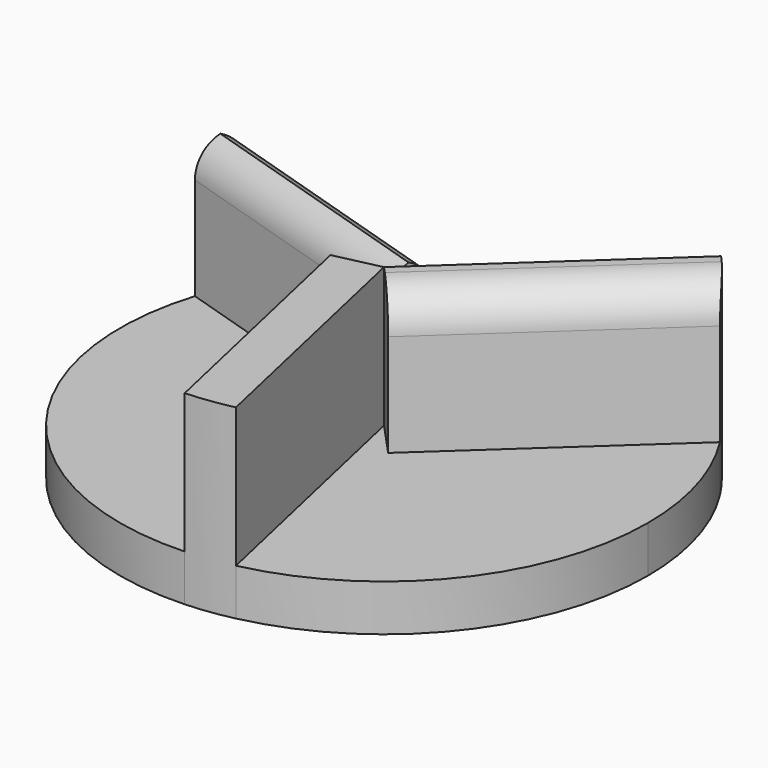
from build123d import *

# Parameters (mm, degrees)
F1_DEPTH      = 25.4
F2_DEPTH      = 6.35
F3_T1_DEPTH   = 61.4532364119
F3_T3_DEPTH   = 60.8896232126
F3_2_T1_DEPTH = 60.8896232126


# Not quite as in the source:
# - a fillet or chamfer that OpenCascade refuses, or shapes differently, is made with other operations: its cross-section is extruded or revolved along the edge and cut away or added


with BuildPart() as f1:
    # F0 (on Top) → F1 (new body)
    with BuildSketch(Plane.XY):
        with BuildLine():
            Line((-34.4173737851, 10.7368634857), (0, 0))
            Line((0, 0), (1.891066931, 6.0618780805))
            Line((1.891066931, 6.0618780805), (-31.9882667756, 16.6308942775))
            ThreePointArc((-31.9882667756, 16.6308942775), (-33.3333492813, 13.737673801), (-34.4173737851, 10.7368634857))
        make_face()
    extrude(amount=F1_DEPTH)

    # F3: fillet of radius 5.08 on 2 edges, made by hand

    # F3_s2 → F3_t1 (cut)
    with BuildSketch(Plane(origin=(-46.541129946, 14.5189973478, 0), x_dir=(0, 0, 1), z_dir=(0.9546264694, -0.2978058159, 0))):
        with BuildLine():
            ThreePointArc((20.32, 0), (23.9121024484, -1.4878975516), (25.4, -5.08))
            Line((25.4, -5.08), (25.4, 0))
            Line((25.4, 0), (20.32, 0))
        make_face()
    extrude(amount=F3_T1_DEPTH, mode=Mode.SUBTRACT)

    # F3_s4 → F3_t3 (cut)
    with BuildSketch(Plane(origin=(12.1237561609, -3.782133862, 0), x_dir=(0, 0, 1), z_dir=(-0.9546264694, 0.2978058159, 0))):
        with BuildLine():
            ThreePointArc((20.32, 6.35), (23.9121024484, 4.8621024484), (25.4, 1.27))
            Line((25.4, 1.27), (25.4, 6.35))
            Line((25.4, 6.35), (20.32, 6.35))
        make_face()
    extrude(amount=F3_T3_DEPTH, mode=Mode.SUBTRACT)


with BuildPart() as f1b:
    # F0 (on Top) → F1, piece 2 (new body)
    with BuildSketch(Plane.XY):
        with BuildLine():
            ThreePointArc((1.5913564558, -36.0180987894), (4.7695001401, -35.7363641714), (7.9102903569, -35.1747517723))
            Line((7.9102903569, -35.1747517723), (0, 0))
            Line((0, 0), (-6.1952738778, -1.3932270377))
            Line((-6.1952738778, -1.3932270377), (1.5913564558, -36.0180987894))
        make_face()
    extrude(amount=F1_DEPTH)


with BuildPart() as f1c:
    # F0 (on Top) → F1, piece 3 (new body)
    with BuildSketch(Plane.XY):
        with BuildLine():
            Line((4.3042069468, -4.6686510427), (30.3969103198, 19.3872045119))
            ThreePointArc((30.3969103198, 19.3872045119), (28.5638491413, 21.9986903703), (26.5070834282, 24.4378882866))
            Line((26.5070834282, 24.4378882866), (0, 0))
            Line((0, 0), (4.3042069468, -4.6686510427))
        make_face()
    extrude(amount=F1_DEPTH)

    # F3#2: fillet of radius 5.08 on 1 edges, made by hand

    # F3_2_s2 → F3_2_t1 (cut)
    with BuildSketch(Plane(origin=(-9.3373020855, -8.6084138936, 0), x_dir=(0, 0, 1), z_dir=(0.7352206367, 0.6778278656, 0))):
        with BuildLine():
            ThreePointArc((20.32, 6.35), (23.9121024484, 4.8621024484), (25.4, 1.27))
            Line((25.4, 1.27), (25.4, 6.35))
            Line((25.4, 6.35), (20.32, 6.35))
        make_face()
    extrude(amount=F3_2_T1_DEPTH, mode=Mode.SUBTRACT)


with BuildPart() as f2:
    # F0 (on Top) → F2 (new body)
    with BuildSketch(Plane.XY):
        with BuildLine():
            ThreePointArc((-34.4173737851, 10.7368634857), (-28.5638491413, -21.9986903703), (1.5913564558, -36.0180987894))
            Line((1.5913564558, -36.0180987894), (-6.1952738778, -1.3932270377))
            Line((-6.1952738778, -1.3932270377), (0, 0))
            Line((0, 0), (-34.4173737851, 10.7368634857))
        make_face()
    extrude(amount=F2_DEPTH)


with BuildPart() as f2b:
    # F0 (on Top) → F2, piece 2 (new body)
    with BuildSketch(Plane.XY):
        with BuildLine():
            ThreePointArc((7.9102903569, -35.1747517723), (28.1516200608, -22.523812815), (36.0532364119, 0))
            ThreePointArc((36.0532364119, 0), (34.6102791792, 10.0977438526), (30.3969103198, 19.3872045119))
            Line((30.3969103198, 19.3872045119), (4.3042069468, -4.6686510427))
            Line((4.3042069468, -4.6686510427), (0, 0))
            Line((0, 0), (7.9102903569, -35.1747517723))
        make_face()
    extrude(amount=F2_DEPTH)


with BuildPart() as f2c:
    # F0 (on Top) → F2, piece 3 (new body)
    with BuildSketch(Plane.XY):
        with BuildLine():
            Line((0, 0), (26.5070834282, 24.4378882866))
            ThreePointArc((26.5070834282, 24.4378882866), (-4.7695001401, 35.7363641714), (-31.9882667756, 16.6308942775))
            Line((-31.9882667756, 16.6308942775), (1.891066931, 6.0618780805))
            Line((1.891066931, 6.0618780805), (0, 0))
        make_face()
    extrude(amount=F2_DEPTH)


solid = Compound([f1.part, f1b.part, f1c.part, f2.part, f2b.part, f2c.part])
